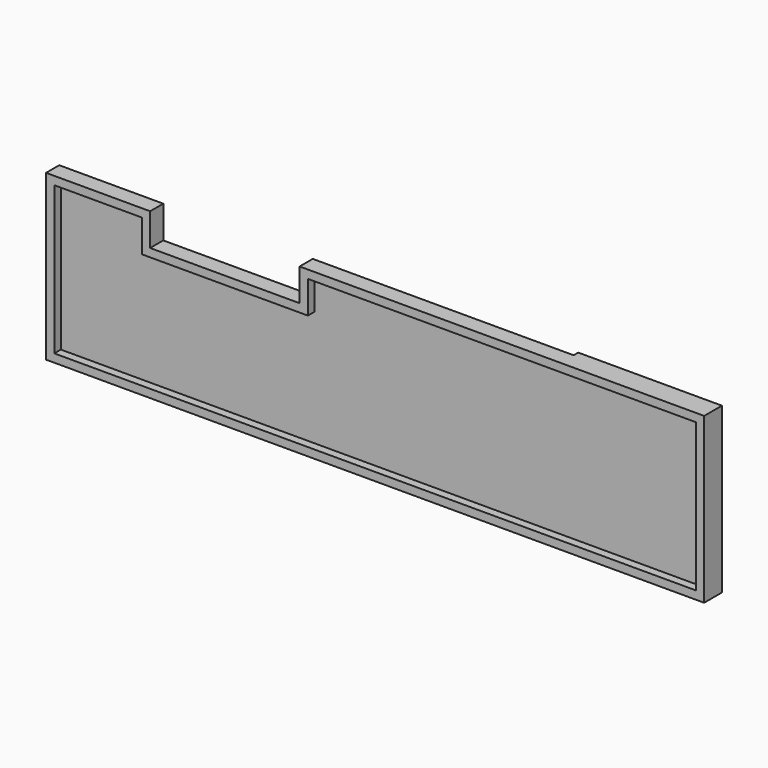
from build123d import *

# Parameters (mm, degrees)
F1_DEPTH = 5.08
F2_T     = -2.54
F3_W     = 3.9589210415
F3_H     = 12.6681532711
F3_W_2   = 146.1344220674
F4_DEPTH = 1.778
F6_DEPTH = 1.778
F7_SIZE  = 12.7
F8_SIZE  = 25.39999


# Not quite as in the source:
# - a fillet or chamfer is up to 0.001 mm smaller than in the source, because OpenCascade refuses the exact size


with BuildPart() as f1:
    # F0 (on Front) → F1 (new body)
    with BuildSketch(Plane.XZ):
        Polygon((104.074490943, -25.4), (104.074490943, 25.4), (-20.8395591676, 25.4), (-20.8395591676, 15.409566462), (-66.9992624521, 15.409566462), (-66.9992624521, 25.4), (-99.125509057, 25.4), (-99.125509057, -25.4), align=None)
    extrude(amount=F1_DEPTH)

    # F2
    f2_openings = [f1.faces().sort_by_distance(p)[0] for p in [
        (4.64404, -5.08, -0.954203),
    ]]
    offset(amount=F2_T, openings=f2_openings, kind=Kind.INTERSECTION)

    # F3 (on face) → F4 (join)
    with BuildSketch(Plane(origin=(0, 0, 0), x_dir=(-1, 0, 0), z_dir=(0, 1, 0))):
        with Locations((101.1049695778, 6.3340766355)):
            Rectangle(F3_W, F3_H)
        with Locations((26.0582980233, 6.3340766355)):
            Rectangle(F3_W_2, F3_H)
    extrude(amount=F4_DEPTH)

    # F5 (on face) → F6 (join)
    with BuildSketch(Plane(origin=(0, 0, 0), x_dir=(-1, 0, 0), z_dir=(0, 1, 0))):
        Polygon((-47.0089130104, 12.6681532711), (-47.0089130104, 25.4), (-104.074490943, 25.4), (-104.074490943, -25.4), (-47.0089130104, -25.4), (-47.0089130104, 0), align=None)
    extrude(amount=F6_DEPTH)

    # F7
    f7_edges = [f1.edges().sort_by_distance(p)[0] for p in [
        (47.008913, 0.889, 25.4),
    ]]
    chamfer(f7_edges, length=F7_SIZE)

    # F8 (size 25.4 in the source; OpenCascade refuses exactly that, so slightly less here)
    f8_edges = [f1.edges().sort_by_distance(p)[0] for p in [
        (47.008913, 0.889, -25.4),
    ]]
    chamfer(f8_edges, length=F8_SIZE)


solid = f1.part
